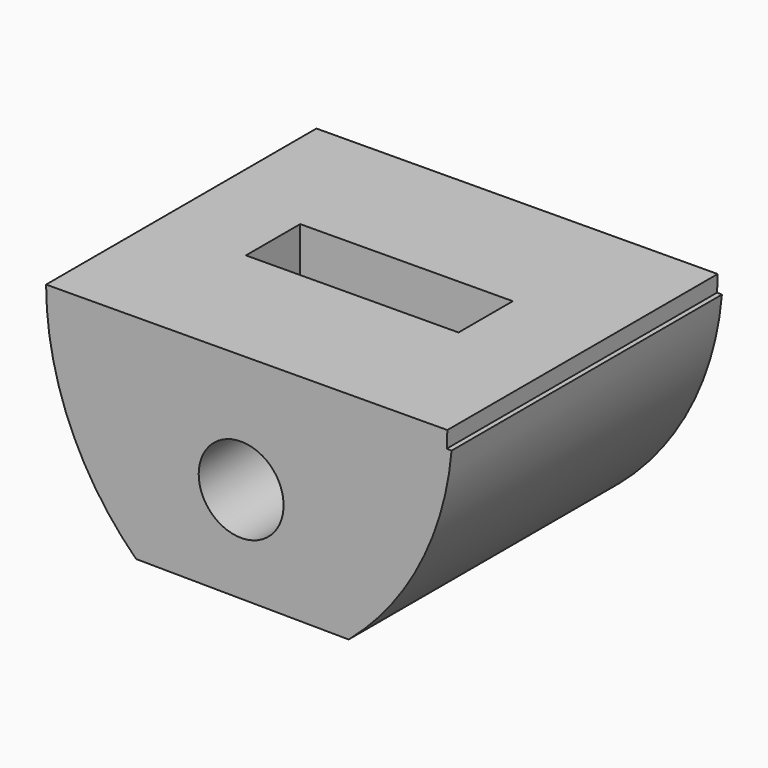
from build123d import *

# Parameters (mm, degrees)
F1_DEPTH = 5.0546
F2_D     = 1.27
F4_DEPTH = 25.4


# Not quite as in the source:
# - a feature names something its author has since deleted; it is built from what else it names


with BuildPart() as f1:
    # F0 (on Front) → F1 (new body)
    with BuildSketch(Plane.XZ):
        Polygon((-45.5380498264, 42.9229369958), (-51.539901644, 42.8869388998), (-45.5468128822, 42.675064641), align=None)
        with BuildLine():
            Line((-45.5468128822, 42.675064641), (-51.539901644, 42.8869388998))
            ThreePointArc((-51.539901644, 42.8869388998), (-51.187813042, 41.162667719), (-50.1936934888, 39.710495621))
            Line((-50.1936934888, 39.710495621), (-47.0142699778, 39.6847687662))
            ThreePointArc((-47.0142699778, 39.6847687662), (-45.9490353675, 41.0264089842), (-45.474623776, 42.6725125324))
            Line((-45.474623776, 42.6725125324), (-45.5468128822, 42.675064641))
        make_face()
    extrude(amount=F1_DEPTH)

    # F2 (through all)
    with Locations(Plane(origin=(0, 0, 0), x_dir=(1, 0, 0), z_dir=(0, 1, 0))):
        with Locations((-48.6222168853, -41.1340259016)):
            Hole(F2_D / 2)

    # F3 (on face) → F4 (cut)
    with BuildSketch(Plane(origin=(0.3180170752, 0, 39.3017713856), x_dir=(0.999967264, 0, -0.0080914079), z_dir=(-0.0080914079, 0, -0.999967264))):
        Polygon((-50.5133641684, 2.0186165348), (-48.9236003704, 2.0186165348), (-47.3338365724, 2.0186165348), (-47.3338365724, 3.0329779256), (-50.5133641684, 3.0329779256), align=None)
    extrude(amount=-F4_DEPTH, mode=Mode.SUBTRACT)


solid = f1.part
